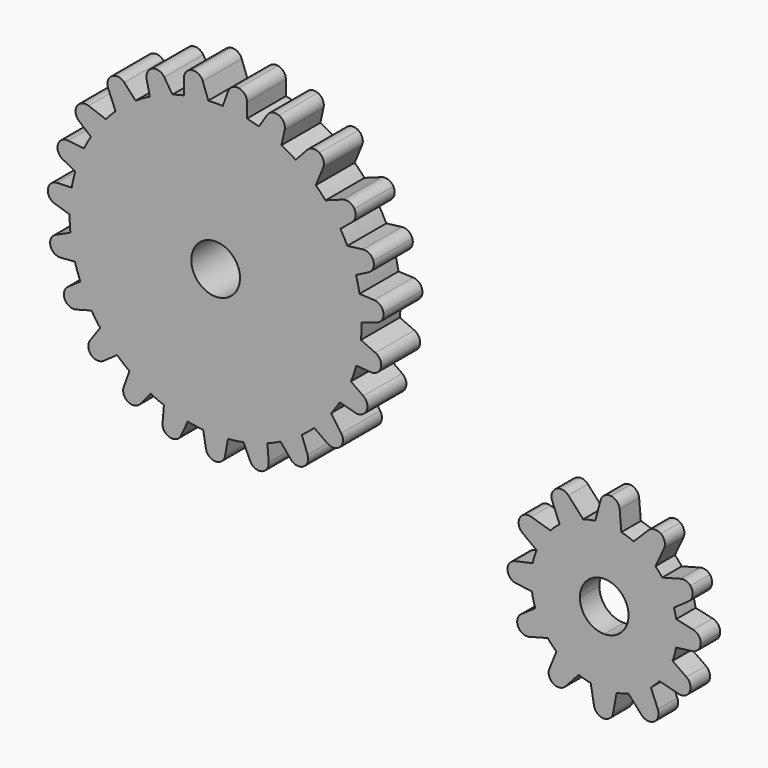
from build123d import *

# Parameters (mm, degrees)
F0_R     = 6.35
F1_DEPTH = 12.7
F3_DEPTH = 6.35


# Not quite as in the source:
# - ends of sketch curves that miss each other by under 0.0002 mm in the source are joined


with BuildPart() as f1:
    # F0 (on Front) → F1 (new body)
    with BuildSketch(Plane.XZ):
        with BuildLine():
            ThreePointArc((-34.9102419123, 17.5729671738), (-34.7547672057, 19.5550047024), (-34.7028952222, 21.5424539336))
            ThreePointArc((-34.7028952222, 21.5424539336), (-34.7029631236, 21.6143850332), (-34.7031668276, 21.6863158763))
            Line((-34.7031668276, 21.6863158763), (-37.8996429288, 20.6795870415))
            Line((-37.8996429288, 20.6795870415), (-38.8881478291, 28.2065023981))
            Line((-38.8881478291, 28.2065023981), (-35.2622454535, 28.047038082))
            ThreePointArc((-35.2622454535, 28.047038082), (-35.6708480799, 30.0759804631), (-36.1890238522, 32.0797412175))
            Line((-36.1890238522, 32.0797412175), (-39.5328523124, 30.3577733792))
            Line((-39.5328523124, 30.3577733792), (-41.7836899824, 37.6079683081))
            Line((-41.7836899824, 37.6079683081), (-38.4556661531, 38.0311729644))
            ThreePointArc((-38.4556661531, 38.0311729644), (-39.3128857232, 39.7091614987), (-40.2520180002, 41.3427163582))
            Line((-40.2520180002, 41.3427163582), (-42.874743432, 39.1419884157))
            Line((-42.874743432, 39.1419884157), (-46.67051729, 45.7164615917))
            Line((-46.67051729, 45.7164615917), (-44.1361986546, 46.6388781391))
            ThreePointArc((-44.1361986546, 46.6388781391), (-45.3794507172, 47.9917392071), (-46.6864795838, 49.2830890057))
            Line((-46.6864795838, 49.2830890057), (-47.6142884848, 47.0420555704))
            Line((-47.6142884848, 47.0420555704), (-54.0176456632, 51.1198752781))
            Line((-54.0176456632, 51.1198752781), (-51.920148722, 53.4096925747))
            ThreePointArc((-51.920148722, 53.4096925747), (-53.748897296, 54.5357132911), (-55.6381867093, 55.5569035347))
            Line((-55.6381867093, 55.5569035347), (-56.4261987077, 52.0361020119))
            Line((-56.4261987077, 52.0361020119), (-63.4339882382, 54.9554311505))
            Line((-63.4339882382, 54.9554311505), (-61.5269208328, 57.9356181485))
            ThreePointArc((-61.5269208328, 57.9356181485), (-63.0677548937, 58.3777229401), (-64.6258220077, 58.7546222881))
            Line((-64.6258220077, 58.7546222881), (-64.6258220077, 55.1074892599))
            Line((-64.6258220077, 55.1074892599), (-72.1020370557, 56.4257476864))
            Line((-72.1020370557, 56.4257476864), (-70.947701025, 59.5972598652))
            ThreePointArc((-70.947701025, 59.5972598652), (-72.8298646656, 59.6424443883), (-74.7119624515, 59.5945952966))
            Line((-74.7119624515, 59.5945952966), (-73.611945077, 56.5723223991))
            Line((-73.611945077, 56.5723223991), (-81.0892134905, 55.2538782358))
            Line((-81.0892134905, 55.2538782358), (-81.0892134905, 58.7304483613))
            ThreePointArc((-81.0892134905, 58.7304483613), (-82.5921118544, 58.3633887089), (-84.0788696115, 57.9356181485))
            Line((-84.0788696115, 57.9356181485), (-82.1718022061, 54.9554311505))
            Line((-82.1718022061, 54.9554311505), (-89.1795917366, 52.0361020119))
            Line((-89.1795917366, 52.0361020119), (-89.967603735, 55.5569035347))
            ThreePointArc((-89.967603735, 55.5569035347), (-91.8568931483, 54.5357132911), (-93.6856417223, 53.4096925747))
            Line((-93.6856417223, 53.4096925747), (-91.5881447811, 51.1198752781))
            Line((-91.5881447811, 51.1198752781), (-97.9915019595, 47.0420555704))
            Line((-97.9915019595, 47.0420555704), (-98.9193108605, 49.2830890057))
            ThreePointArc((-98.9193108605, 49.2830890057), (-100.2263397271, 47.9917392071), (-101.4695917897, 46.6388781391))
            Line((-101.4695917897, 46.6388781391), (-98.9352731543, 45.7164615917))
            Line((-98.9352731543, 45.7164615917), (-102.7310470123, 39.1419884157))
            Line((-102.7310470123, 39.1419884157), (-105.3537724441, 41.3427163582))
            ThreePointArc((-105.3537724441, 41.3427163582), (-106.2929047211, 39.7091614987), (-107.1501242912, 38.0311729644))
            Line((-107.1501242912, 38.0311729644), (-103.8221004619, 37.6079683081))
            Line((-103.8221004619, 37.6079683081), (-106.0729381319, 30.3577733792))
            Line((-106.0729381319, 30.3577733792), (-109.4167665921, 32.0797412175))
            ThreePointArc((-109.4167665921, 32.0797412175), (-109.9349423644, 30.0759804631), (-110.3435449908, 28.047038082))
            Line((-110.3435449908, 28.047038082), (-106.7176426152, 28.2065023981))
            Line((-106.7176426152, 28.2065023981), (-107.7061475155, 20.6795870415))
            Line((-107.7061475155, 20.6795870415), (-110.9026236167, 21.6863158763))
            ThreePointArc((-110.9026236167, 21.6863158763), (-110.854707645, 19.626841412), (-110.695548532, 17.5729671738))
            Line((-110.695548532, 17.5729671738), (-107.69785292, 18.9283214038))
            Line((-107.69785292, 18.9283214038), (-105.8189929076, 11.5729504562))
            Line((-105.8189929076, 11.5729504562), (-109.4987660128, 11.2943776791))
            ThreePointArc((-109.4987660128, 11.2943776791), (-108.8556105251, 9.221264085), (-108.0954397731, 7.1881410235))
            Line((-108.0954397731, 7.1881410235), (-105.2147046971, 9.2065173404))
            Line((-105.2147046971, 9.2065173404), (-102.0043529952, 2.3271831667))
            Line((-102.0043529952, 2.3271831667), (-105.1884891281, 1.4729918741))
            ThreePointArc((-105.1884891281, 1.4729918741), (-104.1087515023, -0.1728255389), (-102.9454542067, -1.760681861))
            Line((-102.9454542067, -1.760681861), (-101.2970690826, 0.5977276055))
            Line((-101.2970690826, 0.5977276055), (-95.9244653315, -4.7657344907))
            Line((-95.9244653315, -4.7657344907), (-98.5090591152, -6.5787682643))
            ThreePointArc((-98.5090591152, -6.5787682643), (-96.9341468953, -7.9413160541), (-95.2871392345, -9.2157770167))
            Line((-95.2871392345, -9.2157770167), (-94.2325988381, -6.3184510895))
            Line((-94.2325988381, -6.3184510895), (-87.658125662, -10.1142249475))
            Line((-87.658125662, -10.1142249475), (-89.734426864, -12.5886643643))
            ThreePointArc((-89.734426864, -12.5886643643), (-88.0370011642, -13.3793446476), (-86.3027767956, -14.0856697541))
            ThreePointArc((-86.3027767956, -14.0856697541), (-83.2302426255, -15.1028790043), (-80.0824621081, -15.8556463651))
            ThreePointArc((-80.0824621081, -15.8556463651), (-78.0770050025, -16.190737901), (-76.0565273803, -16.4183663655))
            ThreePointArc((-76.0565273803, -16.4183663655), (-72.8254583342, -16.5575393854), (-69.5942267157, -16.4221933902))
            ThreePointArc((-69.5942267157, -16.4221933902), (-67.551132252, -16.1938546525), (-65.5233283362, -15.8556463651))
            ThreePointArc((-65.5233283362, -15.8556463651), (-62.3755478188, -15.1028790043), (-59.3030136487, -14.0856697541))
            ThreePointArc((-59.3030136487, -14.0856697541), (-57.5687892801, -13.3793446476), (-55.8713635803, -12.5886643643))
            Line((-55.8713635803, -12.5886643643), (-57.9476647823, -10.1142249475))
            Line((-57.9476647823, -10.1142249475), (-51.3731916062, -6.3184510895))
            Line((-51.3731916062, -6.3184510895), (-50.3186512098, -9.2157770167))
            ThreePointArc((-50.3186512098, -9.2157770167), (-48.671643549, -7.9413160541), (-47.0967313291, -6.5787682643))
            Line((-47.0967313291, -6.5787682643), (-49.6813251128, -4.7657344907))
            Line((-49.6813251128, -4.7657344907), (-44.3087213617, 0.5977276055))
            Line((-44.3087213617, 0.5977276055), (-42.6603362376, -1.760681861))
            ThreePointArc((-42.6603362376, -1.760681861), (-41.497038942, -0.1728255389), (-40.4173013162, 1.4729918741))
            Line((-40.4173013162, 1.4729918741), (-43.6014374491, 2.3271831667))
            Line((-43.6014374491, 2.3271831667), (-40.3910857472, 9.2065173404))
            Line((-40.3910857472, 9.2065173404), (-37.5103506712, 7.1881410235))
            ThreePointArc((-37.5103506712, 7.1881410235), (-36.7501799192, 9.221264085), (-36.1070244315, 11.2943776791))
            Line((-36.1070244315, 11.2943776791), (-39.7867975367, 11.5729504562))
            Line((-39.7867975367, 11.5729504562), (-37.9079375243, 18.9283214038))
            Line((-37.9079375243, 18.9283214038), (-34.9102419123, 17.5729671738))
        make_face()
        with Locations((-72.8028952222, 21.5424539336)):
            Circle(F0_R, mode=Mode.SUBTRACT)
        with BuildLine():
            Line((-37.8996429288, 20.6795870415), (-34.7031668276, 21.6863158763))
            ThreePointArc((-34.7031668276, 21.6863158763), (-34.8492208425, 24.8784097313), (-35.2622454535, 28.047038082))
            Line((-35.2622454535, 28.047038082), (-38.8881478291, 28.2065023981))
            Line((-38.8881478291, 28.2065023981), (-37.8996429288, 20.6795870415))
        make_face()
        with BuildLine():
            ThreePointArc((-35.2622454535, 28.047038082), (-34.8492208425, 24.8784097313), (-34.7031668276, 21.6863158763))
            Line((-34.7031668276, 21.6863158763), (-30.7899816117, 22.9187719524))
            ThreePointArc((-30.7899816117, 22.9187719524), (-29.4112241553, 23.9760340856), (-29.0346296669, 25.6721920773))
            ThreePointArc((-29.0346296669, 25.6721920773), (-29.836410615, 27.2135926365), (-31.4414052089, 27.8790005528))
            Line((-31.4414052089, 27.8790005528), (-35.2622454535, 28.047038082))
        make_face()
        with BuildLine():
            Line((-31.1159582959, 15.857449985), (-34.9102419123, 17.5729671738))
            ThreePointArc((-34.9102419123, 17.5729671738), (-35.3767392162, 14.4085316873), (-36.1070244315, 11.2943776791))
            Line((-36.1070244315, 11.2943776791), (-32.3541248925, 11.0102689537))
            ThreePointArc((-32.3541248925, 11.0102689537), (-30.6812444479, 11.4795730766), (-29.7014065548, 12.9143877143))
            ThreePointArc((-29.7014065548, 12.9143877143), (-29.8730887811, 14.643345084), (-31.1159582959, 15.857449985))
        make_face()
        with BuildLine():
            ThreePointArc((-36.1070244315, 11.2943776791), (-35.3767392162, 14.4085316873), (-34.9102419123, 17.5729671738))
            Line((-34.9102419123, 17.5729671738), (-37.9079375243, 18.9283214038))
            Line((-37.9079375243, 18.9283214038), (-39.7867975367, 11.5729504562))
            Line((-39.7867975367, 11.5729504562), (-36.1070244315, 11.2943776791))
        make_face()
        with BuildLine():
            Line((-39.5328523124, 30.3577733792), (-36.1890238522, 32.0797412175))
            ThreePointArc((-36.1890238522, 32.0797412175), (-37.1977786118, 35.1028990281), (-38.4556661531, 38.0311729644))
            Line((-38.4556661531, 38.0311729644), (-41.7836899824, 37.6079683081))
            Line((-41.7836899824, 37.6079683081), (-39.5328523124, 30.3577733792))
        make_face()
        with BuildLine():
            ThreePointArc((-38.4556661531, 38.0311729644), (-37.1977786118, 35.1028990281), (-36.1890238522, 32.0797412175))
            Line((-36.1890238522, 32.0797412175), (-32.9059961539, 33.7703985511))
            ThreePointArc((-32.9059961539, 33.7703985511), (-31.7265399954, 35.0461957574), (-31.643090796, 36.7816529228))
            ThreePointArc((-31.643090796, 36.7816529228), (-32.6946947308, 38.1647283138), (-34.3892956008, 38.5482687065))
            Line((-34.3892956008, 38.5482687065), (-38.4556661531, 38.0311729644))
        make_face()
        with BuildLine():
            Line((-34.2864336087, 4.9293155241), (-37.5103506712, 7.1881410235))
            ThreePointArc((-37.5103506712, 7.1881410235), (-38.8433849386, 4.26930537), (-40.4173013162, 1.4729918741))
            Line((-40.4173013162, 1.4729918741), (-36.4020517039, 0.3958421817))
            ThreePointArc((-36.4020517039, 0.3958421817), (-34.6711564476, 0.5467625362), (-33.4422234889, 1.7749722596))
            ThreePointArc((-33.4422234889, 1.7749722596), (-33.2902851196, 3.5057764382), (-34.2864336087, 4.9293155241))
        make_face()
        with BuildLine():
            ThreePointArc((-40.4173013162, 1.4729918741), (-38.8433849386, 4.26930537), (-37.5103506712, 7.1881410235))
            Line((-37.5103506712, 7.1881410235), (-40.3910857472, 9.2065173404))
            Line((-40.3910857472, 9.2065173404), (-43.6014374491, 2.3271831667))
            Line((-43.6014374491, 2.3271831667), (-40.4173013162, 1.4729918741))
        make_face()
        with BuildLine():
            Line((-42.874743432, 39.1419884157), (-40.2520180002, 41.3427163582))
            ThreePointArc((-40.2520180002, 41.3427163582), (-42.0797741637, 44.0746493976), (-44.1361986546, 46.6388781391))
            Line((-44.1361986546, 46.6388781391), (-46.67051729, 45.7164615917))
            Line((-46.67051729, 45.7164615917), (-42.874743432, 39.1419884157))
        make_face()
        with BuildLine():
            ThreePointArc((-44.1361986546, 46.6388781391), (-42.0797741637, 44.0746493976), (-40.2520180002, 41.3427163582))
            Line((-40.2520180002, 41.3427163582), (-37.1646935203, 43.9332891906))
            ThreePointArc((-37.1646935203, 43.9332891906), (-36.2959623563, 45.4379757048), (-36.5976695233, 47.1490420761))
            ThreePointArc((-36.5976695233, 47.1490420761), (-37.9286418178, 48.2658594847), (-39.6661041459, 48.2658594847))
            Line((-39.6661041459, 48.2658594847), (-44.1361986546, 46.6388781391))
        make_face()
        with BuildLine():
            Line((-40.0385172453, -5.5118214706), (-42.6603362376, -1.760681861))
            ThreePointArc((-42.6603362376, -1.760681861), (-44.7748119678, -4.265229982), (-47.0967313291, -6.5787682643))
            Line((-47.0967313291, -6.5787682643), (-43.5790569647, -9.0463368499))
            ThreePointArc((-43.5790569647, -9.0463368499), (-41.9011807432, -9.4974540487), (-40.3258804416, -8.7645118264))
            ThreePointArc((-40.3258804416, -8.7645118264), (-39.5902580888, -7.1904635022), (-40.0385172453, -5.5118214706))
        make_face()
        with BuildLine():
            ThreePointArc((-47.0967313291, -6.5787682643), (-44.7748119678, -4.265229982), (-42.6603362376, -1.760681861))
            Line((-42.6603362376, -1.760681861), (-44.3087213617, 0.5977276055))
            Line((-44.3087213617, 0.5977276055), (-49.6813251128, -4.7657344907))
            Line((-49.6813251128, -4.7657344907), (-47.0967313291, -6.5787682643))
        make_face()
        with BuildLine():
            Line((-47.6142884848, 47.0420555704), (-46.6864795838, 49.2830890057))
            ThreePointArc((-46.6864795838, 49.2830890057), (-49.2129074162, 51.461051416), (-51.920148722, 53.4096925747))
            Line((-51.920148722, 53.4096925747), (-54.0176456632, 51.1198752781))
            Line((-54.0176456632, 51.1198752781), (-47.6142884848, 47.0420555704))
        make_face()
        with BuildLine():
            ThreePointArc((-51.920148722, 53.4096925747), (-49.2129074162, 51.461051416), (-46.6864795838, 49.2830890057))
            Line((-46.6864795838, 49.2830890057), (-44.7629890646, 53.9290959164))
            ThreePointArc((-44.7629890646, 53.9290959164), (-44.6875045379, 55.664917747), (-45.7454448011, 57.0431549331))
            ThreePointArc((-45.7454448011, 57.0431549331), (-47.4417860472, 57.4189138315), (-48.9827941123, 56.6163744339))
            Line((-48.9827941123, 56.6163744339), (-51.920148722, 53.4096925747))
        make_face()
        with BuildLine():
            Line((-48.8237937133, -13.3228642336), (-50.3186512098, -9.2157770167))
            ThreePointArc((-50.3186512098, -9.2157770167), (-53.0229828141, -11.0207932191), (-55.8713635803, -12.5886643643))
            Line((-55.8713635803, -12.5886643643), (-53.1563640074, -15.8242748592))
            ThreePointArc((-53.1563640074, -15.8242748592), (-51.6516774932, -16.6930060232), (-49.9406111219, -16.3912988562))
            ThreePointArc((-49.9406111219, -16.3912988562), (-48.8237937133, -15.0603265617), (-48.8237937133, -13.3228642336))
        make_face()
        with BuildLine():
            ThreePointArc((-55.8713635803, -12.5886643643), (-53.0229828141, -11.0207932191), (-50.3186512098, -9.2157770167))
            Line((-50.3186512098, -9.2157770167), (-51.3731916062, -6.3184510895))
            Line((-51.3731916062, -6.3184510895), (-57.9476647823, -10.1142249475))
            Line((-57.9476647823, -10.1142249475), (-55.8713635803, -12.5886643643))
        make_face()
        with BuildLine():
            Line((-56.4261987077, 52.0361020119), (-55.6381867093, 55.5569035347))
            ThreePointArc((-55.6381867093, 55.5569035347), (-58.5329028679, 56.8691763716), (-61.5269208328, 57.9356181485))
            Line((-61.5269208328, 57.9356181485), (-63.4339882382, 54.9554311505))
            Line((-63.4339882382, 54.9554311505), (-56.4261987077, 52.0361020119))
        make_face()
        with BuildLine():
            ThreePointArc((-61.5269208328, 57.9356181485), (-58.5329028679, 56.8691763716), (-55.6381867093, 55.5569035347))
            Line((-55.6381867093, 55.5569035347), (-54.7981656804, 59.3100790239))
            ThreePointArc((-54.7981656804, 59.3100790239), (-55.0214679679, 61.0331319627), (-56.3000845242, 62.2095311481))
            ThreePointArc((-56.3000845242, 62.2095311481), (-58.0357344825, 62.2888255062), (-59.4162909558, 61.2339135831))
            Line((-59.4162909558, 61.2339135831), (-61.5269208328, 57.9356181485))
        make_face()
        with BuildLine():
            Line((-58.9548245325, -18.3537802527), (-59.3030136487, -14.0856697541))
            ThreePointArc((-59.3030136487, -14.0856697541), (-62.3755478188, -15.1028790043), (-65.5233283362, -15.8556463651))
            Line((-65.5233283362, -15.8556463651), (-63.7946929451, -19.6202297071))
            ThreePointArc((-63.7946929451, -19.6202297071), (-62.5733513004, -20.8559885544), (-60.8434188448, -21.017571476))
            ThreePointArc((-60.8434188448, -21.017571476), (-59.4143522649, -20.0293725673), (-58.9548245325, -18.3537802527))
        make_face()
        with BuildLine():
            Line((-64.6258220077, 55.1074892599), (-64.6258220077, 58.7546222881))
            ThreePointArc((-64.6258220077, 58.7546222881), (-67.7690987546, 59.308455749), (-70.947701025, 59.5972598652))
            Line((-70.947701025, 59.5972598652), (-72.1020370557, 56.4257476864))
            Line((-72.1020370557, 56.4257476864), (-64.6258220077, 55.1074892599))
        make_face()
        with BuildLine():
            ThreePointArc((-70.947701025, 59.5972598652), (-67.7690987546, 59.308455749), (-64.6258220077, 58.7546222881))
            Line((-64.6258220077, 58.7546222881), (-64.6258220077, 62.561430037))
            ThreePointArc((-64.6258220077, 62.561430037), (-65.2200691221, 64.1941105656), (-66.7247556364, 65.0628417297))
            ThreePointArc((-66.7247556364, 65.0628417297), (-68.4358199059, 64.761134192), (-69.5526391627, 63.4301608305))
            Line((-69.5526391627, 63.4301608305), (-70.947701025, 59.5972598652))
        make_face()
        with BuildLine():
            Line((-70.3236177997, -20.5587757844), (-69.5942267157, -16.4221933902))
            ThreePointArc((-69.5942267157, -16.4221933902), (-72.8254583342, -16.5575393854), (-76.0565273803, -16.4183663655))
            Line((-76.0565273803, -16.4183663655), (-75.3264614886, -20.5587757844))
            ThreePointArc((-75.3264614886, -20.5587757844), (-74.4577303246, -22.0634622987), (-72.825049796, -22.6577094132))
            ThreePointArc((-72.825049796, -22.6577094132), (-71.1923489638, -22.0634622987), (-70.3236177997, -20.5587757844))
        make_face()
        with BuildLine():
            Line((-73.611945077, 56.5723223991), (-74.7119624515, 59.5945952966))
            ThreePointArc((-74.7119624515, 59.5945952966), (-77.9188661802, 59.297411769), (-81.0892134905, 58.7304483613))
            Line((-81.0892134905, 58.7304483613), (-81.0892134905, 55.2538782358))
            Line((-81.0892134905, 55.2538782358), (-73.611945077, 56.5723223991))
        make_face()
        with BuildLine():
            ThreePointArc((-81.0892134905, 58.7304483613), (-77.9188661802, 59.297411769), (-74.7119624515, 59.5945952966))
            Line((-74.7119624515, 59.5945952966), (-76.1623742386, 63.5795689305))
            ThreePointArc((-76.1623742386, 63.5795689305), (-77.2791934954, 64.9105422921), (-78.9902598666, 65.2122494591))
            ThreePointArc((-78.9902598666, 65.2122494591), (-80.494966376, 64.3435147694), (-81.0892134905, 62.7108342408))
            Line((-81.0892134905, 62.7108342408), (-81.0892134905, 58.7304483613))
        make_face()
        with BuildLine():
            Line((-81.8110974992, -19.6202297071), (-80.0824621081, -15.8556463651))
            ThreePointArc((-80.0824621081, -15.8556463651), (-83.2302426255, -15.1028790043), (-86.3027767956, -14.0856697541))
            Line((-86.3027767956, -14.0856697541), (-86.6509659118, -18.3537802527))
            ThreePointArc((-86.6509659118, -18.3537802527), (-86.1914381794, -20.0293725673), (-84.7623695349, -21.0175720162))
            ThreePointArc((-84.7623695349, -21.0175720162), (-83.0324391439, -20.8559885544), (-81.8110974992, -19.6202297071))
        make_face()
        with BuildLine():
            Line((-82.1718022061, 54.9554311505), (-84.0788696115, 57.9356181485))
            ThreePointArc((-84.0788696115, 57.9356181485), (-87.0728875764, 56.8691763716), (-89.967603735, 55.5569035347))
            Line((-89.967603735, 55.5569035347), (-89.1795917366, 52.0361020119))
            Line((-89.1795917366, 52.0361020119), (-82.1718022061, 54.9554311505))
        make_face()
        with BuildLine():
            ThreePointArc((-89.967603735, 55.5569035347), (-87.0728875764, 56.8691763716), (-84.0788696115, 57.9356181485))
            Line((-84.0788696115, 57.9356181485), (-86.1894994885, 61.2339135831))
            ThreePointArc((-86.1894994885, 61.2339135831), (-87.5700559618, 62.2888255062), (-89.3057078901, 62.2095303274))
            ThreePointArc((-89.3057078901, 62.2095303274), (-90.5843224764, 61.0331319627), (-90.8076247639, 59.3100790239))
            Line((-90.8076247639, 59.3100790239), (-89.967603735, 55.5569035347))
        make_face()
        with BuildLine():
            Line((-92.4494264369, -15.8242748592), (-89.734426864, -12.5886643643))
            ThreePointArc((-89.734426864, -12.5886643643), (-92.5828076302, -11.0207932191), (-95.2871392345, -9.2157770167))
            Line((-95.2871392345, -9.2157770167), (-96.781996731, -13.3228642336))
            ThreePointArc((-96.781996731, -13.3228642336), (-96.781996731, -15.0603265617), (-95.6651774742, -16.3912999233))
            ThreePointArc((-95.6651774742, -16.3912999233), (-93.9541129511, -16.6930060232), (-92.4494264369, -15.8242748592))
        make_face()
        with BuildLine():
            ThreePointArc((-95.2871392345, -9.2157770167), (-92.5828076302, -11.0207932191), (-89.734426864, -12.5886643643))
            Line((-89.734426864, -12.5886643643), (-87.658125662, -10.1142249475))
            Line((-87.658125662, -10.1142249475), (-94.2325988381, -6.3184510895))
            Line((-94.2325988381, -6.3184510895), (-95.2871392345, -9.2157770167))
        make_face()
        with BuildLine():
            Line((-91.5881447811, 51.1198752781), (-93.6856417223, 53.4096925747))
            ThreePointArc((-93.6856417223, 53.4096925747), (-96.3928830281, 51.461051416), (-98.9193108605, 49.2830890057))
            Line((-98.9193108605, 49.2830890057), (-97.9915019595, 47.0420555704))
            Line((-97.9915019595, 47.0420555704), (-91.5881447811, 51.1198752781))
        make_face()
        with BuildLine():
            ThreePointArc((-98.9193108605, 49.2830890057), (-96.3928830281, 51.461051416), (-93.6856417223, 53.4096925747))
            Line((-93.6856417223, 53.4096925747), (-96.622996332, 56.6163744339))
            ThreePointArc((-96.622996332, 56.6163744339), (-98.1640043971, 57.4189138315), (-99.8603474433, 57.0431537868))
            ThreePointArc((-99.8603474433, 57.0431537868), (-100.9182859064, 55.664917747), (-100.8428013797, 53.9290959164))
            Line((-100.8428013797, 53.9290959164), (-98.9193108605, 49.2830890057))
        make_face()
        with BuildLine():
            Line((-102.0267334796, -9.0463368499), (-98.5090591152, -6.5787682643))
            ThreePointArc((-98.5090591152, -6.5787682643), (-100.8309784765, -4.265229982), (-102.9454542067, -1.760681861))
            Line((-102.9454542067, -1.760681861), (-105.567273199, -5.5118214706))
            ThreePointArc((-105.567273199, -5.5118214706), (-106.0155323555, -7.1904635022), (-105.2799084923, -8.7645133341))
            ThreePointArc((-105.2799084923, -8.7645133341), (-103.7046097011, -9.4974540487), (-102.0267334796, -9.0463368499))
        make_face()
        with BuildLine():
            ThreePointArc((-102.9454542067, -1.760681861), (-100.8309784765, -4.265229982), (-98.5090591152, -6.5787682643))
            Line((-98.5090591152, -6.5787682643), (-95.9244653315, -4.7657344907))
            Line((-95.9244653315, -4.7657344907), (-101.2970690826, 0.5977276055))
            Line((-101.2970690826, 0.5977276055), (-102.9454542067, -1.760681861))
        make_face()
        with BuildLine():
            Line((-98.9352731543, 45.7164615917), (-101.4695917897, 46.6388781391))
            ThreePointArc((-101.4695917897, 46.6388781391), (-103.5260162806, 44.0746493976), (-105.3537724441, 41.3427163582))
            Line((-105.3537724441, 41.3427163582), (-102.7310470123, 39.1419884157))
            Line((-102.7310470123, 39.1419884157), (-98.9352731543, 45.7164615917))
        make_face()
        with BuildLine():
            ThreePointArc((-105.3537724441, 41.3427163582), (-103.5260162806, 44.0746493976), (-101.4695917897, 46.6388781391))
            Line((-101.4695917897, 46.6388781391), (-105.9396862984, 48.2658594847))
            ThreePointArc((-105.9396862984, 48.2658594847), (-107.6771486265, 48.2658594847), (-109.008121988, 47.1490402279))
            ThreePointArc((-109.008121988, 47.1490402279), (-109.309828088, 45.4379757048), (-108.441096924, 43.9332891906))
            Line((-108.441096924, 43.9332891906), (-105.3537724441, 41.3427163582))
        make_face()
        with BuildLine():
            Line((-109.2037387404, 0.3958421817), (-105.1884891281, 1.4729918741))
            ThreePointArc((-105.1884891281, 1.4729918741), (-106.7624055057, 4.26930537), (-108.0954397731, 7.1881410235))
            Line((-108.0954397731, 7.1881410235), (-111.3193568356, 4.9293155241))
            ThreePointArc((-111.3193568356, 4.9293155241), (-112.3155053247, 3.5057764382), (-112.1635660529, 1.7749703256))
            ThreePointArc((-112.1635660529, 1.7749703256), (-110.9346339967, 0.5467625362), (-109.2037387404, 0.3958421817))
        make_face()
        with BuildLine():
            ThreePointArc((-108.0954397731, 7.1881410235), (-106.7624055057, 4.26930537), (-105.1884891281, 1.4729918741))
            Line((-105.1884891281, 1.4729918741), (-102.0043529952, 2.3271831667))
            Line((-102.0043529952, 2.3271831667), (-105.2147046971, 9.2065173404))
            Line((-105.2147046971, 9.2065173404), (-108.0954397731, 7.1881410235))
        make_face()
        with BuildLine():
            Line((-103.8221004619, 37.6079683081), (-107.1501242912, 38.0311729644))
            ThreePointArc((-107.1501242912, 38.0311729644), (-108.4080118325, 35.1028990281), (-109.4167665921, 32.0797412175))
            Line((-109.4167665921, 32.0797412175), (-106.0729381319, 30.3577733792))
            Line((-106.0729381319, 30.3577733792), (-103.8221004619, 37.6079683081))
        make_face()
        with BuildLine():
            ThreePointArc((-109.4167665921, 32.0797412175), (-108.4080118325, 35.1028990281), (-107.1501242912, 38.0311729644))
            Line((-107.1501242912, 38.0311729644), (-111.2164948435, 38.5482687065))
            ThreePointArc((-111.2164948435, 38.5482687065), (-112.9110957135, 38.1647283138), (-113.962700281, 36.7816508846))
            ThreePointArc((-113.962700281, 36.7816508846), (-113.8792504489, 35.0461957574), (-112.6997942904, 33.7703985511))
            Line((-112.6997942904, 33.7703985511), (-109.4167665921, 32.0797412175))
        make_face()
        with BuildLine():
            Line((-113.2516655518, 11.0102689537), (-109.4987660128, 11.2943776791))
            ThreePointArc((-109.4987660128, 11.2943776791), (-110.2290512281, 14.4085316873), (-110.695548532, 17.5729671738))
            Line((-110.695548532, 17.5729671738), (-114.4898321484, 15.857449985))
            ThreePointArc((-114.4898321484, 15.857449985), (-115.7327016632, 14.643345084), (-115.9043833613, 12.9143856466))
            ThreePointArc((-115.9043833613, 12.9143856466), (-114.9245459964, 11.4795730766), (-113.2516655518, 11.0102689537))
        make_face()
        with BuildLine():
            ThreePointArc((-110.695548532, 17.5729671738), (-110.2290512281, 14.4085316873), (-109.4987660128, 11.2943776791))
            Line((-109.4987660128, 11.2943776791), (-105.8189929076, 11.5729504562))
            Line((-105.8189929076, 11.5729504562), (-107.69785292, 18.9283214038))
            Line((-107.69785292, 18.9283214038), (-110.695548532, 17.5729671738))
        make_face()
        with BuildLine():
            Line((-106.7176426152, 28.2065023981), (-110.3435449908, 28.047038082))
            ThreePointArc((-110.3435449908, 28.047038082), (-110.7565696018, 24.8784097313), (-110.9026236167, 21.6863158763))
            Line((-110.9026236167, 21.6863158763), (-107.7061475155, 20.6795870415))
            Line((-107.7061475155, 20.6795870415), (-106.7176426152, 28.2065023981))
        make_face()
        with BuildLine():
            ThreePointArc((-110.9026236167, 21.6863158763), (-110.7565696018, 24.8784097313), (-110.3435449908, 28.047038082))
            Line((-110.3435449908, 28.047038082), (-114.1643852354, 27.8790005528))
            ThreePointArc((-114.1643852354, 27.8790005528), (-115.7693798293, 27.2135926365), (-116.5711610553, 25.6721899613))
            ThreePointArc((-116.5711610553, 25.6721899613), (-116.194566289, 23.9760340856), (-114.8158088326, 22.9187719524))
            Line((-114.8158088326, 22.9187719524), (-110.9026236167, 21.6863158763))
        make_face()
    extrude(amount=F1_DEPTH)


with BuildPart() as f3:
    # F2 (on Front) → F3 (new body)
    with BuildSketch(Plane.XZ):
        with BuildLine():
            Line((39.2386662279, -27.221067247), (42.5388315106, -27.221067247))
            ThreePointArc((42.5388315106, -27.221067247), (42.4712083716, -25.6173625646), (42.2688190478, -24.0250434511))
            Line((42.2688190478, -24.0250434511), (39.4114386524, -23.3873699688))
            Line((39.4114386524, -23.3873699688), (39.2386662279, -27.221067247))
        make_face()
        with BuildLine():
            ThreePointArc((42.2688190478, -24.0250434511), (42.4712083716, -25.6173625646), (42.5388315106, -27.221067247))
            ThreePointArc((42.5388315106, -27.221067247), (42.4650633594, -28.8959179328), (42.2443302172, -30.5577974229))
            Line((42.2443302172, -30.5577974229), (46.4611879954, -30.0086556109))
            ThreePointArc((46.4611879954, -30.0086556109), (48.0034600385, -29.2085479391), (48.6706096692, -27.6042765431))
            ThreePointArc((48.6706096692, -27.6042765431), (48.1504700645, -25.9464999706), (46.6864204734, -25.0109070375))
            Line((46.6864204734, -25.0109070375), (42.2688190478, -24.0250434511))
        make_face()
        with BuildLine():
            ThreePointArc((42.2443302172, -30.5577974229), (42.4650633594, -28.8959179328), (42.5388315106, -27.221067247))
            Line((42.5388315106, -27.221067247), (39.2386662279, -27.221067247))
            Line((39.2386662279, -27.221067247), (39.0696588809, -30.9712201329))
            Line((39.0696588809, -30.9712201329), (42.2443302172, -30.5577974229))
        make_face()
        with BuildLine():
            Line((39.4114386524, -23.3873699688), (42.2688190478, -24.0250434511))
            ThreePointArc((42.2688190478, -24.0250434511), (42.0144891046, -22.7823162165), (41.6780192026, -21.5592697315))
            Line((41.6780192026, -21.5592697315), (39.3024932084, -23.217564621))
            Line((39.3024932084, -23.217564621), (36.1040258476, -16.3326969196))
            Line((36.1040258476, -16.3326969196), (38.6295404081, -15.6598634135))
            ThreePointArc((38.6295404081, -15.6598634135), (37.7754241148, -14.6196478126), (36.8499909676, -13.6423368953))
            Line((36.8499909676, -13.6423368953), (35.9346611892, -15.6009121348))
            Line((35.9346611892, -15.6009121348), (29.7197392831, -11.2412857258))
            Line((29.7197392831, -11.2412857258), (31.1736239134, -9.7898749262))
            ThreePointArc((31.1736239134, -9.7898749262), (29.590831745, -9.1747908128), (27.9595541548, -8.7030992419))
            Line((27.9595541548, -8.7030992419), (28.1592660179, -11.0084230784))
            Line((28.1592660179, -11.0084230784), (23.4888315106, -10.5958054377))
            Line((23.4888315106, -10.5958054377), (23.4888315106, -20.871067247))
            ThreePointArc((23.4888315106, -20.871067247), (27.9789595711, -22.7309391865), (29.8388315106, -27.221067247))
            Line((29.8388315106, -27.221067247), (39.2386662279, -27.221067247))
            Line((39.2386662279, -27.221067247), (39.4114386524, -23.3873699688))
        make_face()
        with BuildLine():
            ThreePointArc((41.3188553639, -33.9287307292), (41.8590768297, -32.2645369769), (42.2443302172, -30.5577974229))
            Line((42.2443302172, -30.5577974229), (39.0696588809, -30.9712201329))
            Line((39.0696588809, -30.9712201329), (39.2386662279, -27.221067247))
            Line((39.2386662279, -27.221067247), (29.8388315106, -27.221067247))
            ThreePointArc((29.8388315106, -27.221067247), (27.9789595711, -31.7111953075), (23.4888315106, -33.571067247))
            Line((23.4888315106, -33.571067247), (23.4888315106, -43.5467305829))
            Line((23.4888315106, -43.5467305829), (27.1324330255, -43.5498330739))
            Line((27.1324330255, -43.5498330739), (26.6984757495, -45.9987317413))
            ThreePointArc((26.6984757495, -45.9987317413), (28.2725179937, -45.6606671242), (29.8123945292, -45.1909044958))
            Line((29.8123945292, -45.1909044958), (28.2482940818, -43.4686322552))
            Line((28.2482940818, -43.4686322552), (34.6690657771, -39.4182881266))
            Line((34.6690657771, -39.4182881266), (35.6706278235, -41.8671021572))
            ThreePointArc((35.6706278235, -41.8671021572), (36.8326720529, -40.8168173029), (37.9045036776, -39.6746167801))
            Line((37.9045036776, -39.6746167801), (35.6145713384, -39.0631206306))
            Line((35.6145713384, -39.0631206306), (38.817038387, -32.1801124564))
            Line((38.817038387, -32.1801124564), (41.3188553639, -33.9287307292))
        make_face()
        with BuildLine():
            Line((39.3024932084, -23.217564621), (41.6780192026, -21.5592697315))
            ThreePointArc((41.6780192026, -21.5592697315), (40.4128159821, -18.475711359), (38.6295404081, -15.6598634135))
            Line((38.6295404081, -15.6598634135), (36.1040258476, -16.3326969196))
            Line((36.1040258476, -16.3326969196), (39.3024932084, -23.217564621))
        make_face()
        with BuildLine():
            ThreePointArc((38.6295404081, -15.6598634135), (40.4128159821, -18.475711359), (41.6780192026, -21.5592697315))
            Line((41.6780192026, -21.5592697315), (45.414522316, -18.9509109794))
            ThreePointArc((45.414522316, -18.9509109794), (46.5152556137, -17.179281474), (46.0014613402, -15.157821521))
            ThreePointArc((46.0014613402, -15.157821521), (44.7656661613, -14.3817317553), (43.306735988, -14.4137910486))
            Line((43.306735988, -14.4137910486), (38.6295404081, -15.6598634135))
        make_face()
        with BuildLine():
            Line((44.9265874631, -36.4503165729), (41.3188553639, -33.9287307292))
            ThreePointArc((41.3188553639, -33.9287307292), (39.8656452906, -36.9525866769), (37.9045036776, -39.6746167801))
            Line((37.9045036776, -39.6746167801), (42.8161653454, -40.9862110774))
            ThreePointArc((42.8161653454, -40.9862110774), (44.5468865364, -40.8333075107), (45.7744113691, -39.6036904457))
            ThreePointArc((45.7744113691, -39.6036904457), (45.9243664317, -37.8727133077), (44.9265874631, -36.4503165729))
        make_face()
        with BuildLine():
            ThreePointArc((37.9045036776, -39.6746167801), (39.8656452906, -36.9525866769), (41.3188553639, -33.9287307292))
            Line((41.3188553639, -33.9287307292), (38.817038387, -32.1801124564))
            Line((38.817038387, -32.1801124564), (35.6145713384, -39.0631206306))
            Line((35.6145713384, -39.0631206306), (37.9045036776, -39.6746167801))
        make_face()
        with BuildLine():
            ThreePointArc((17.1388315106, -27.221067247), (18.9987034501, -22.7309391865), (23.4888315106, -20.871067247))
            Line((23.4888315106, -20.871067247), (23.4888315106, -10.5958054377))
            Line((23.4888315106, -10.5958054377), (20.5971725602, -10.3403368102))
            Line((20.5971725602, -10.3403368102), (21.1413713275, -8.3162548785))
            ThreePointArc((21.1413713275, -8.3162548785), (19.5588049741, -8.5808582508), (18.0041193214, -8.9777004469))
            Line((18.0041193214, -8.9777004469), (19.1701500942, -10.2566665492))
            Line((19.1701500942, -10.2566665492), (12.7572274857, -14.3194267367))
            Line((12.7572274857, -14.3194267367), (11.8582732366, -12.1335686394))
            ThreePointArc((11.8582732366, -12.1335686394), (10.614507997, -13.1799029767), (9.4644620612, -14.3284506954))
            Line((9.4644620612, -14.3284506954), (11.5601212245, -14.9575260151))
            Line((11.5601212245, -14.9575260151), (8.1480631412, -21.7390786662))
            Line((8.1480631412, -21.7390786662), (5.8500100327, -20.0256189029))
            ThreePointArc((5.8500100327, -20.0256189029), (5.2671352493, -21.6647838346), (4.8362293039, -23.3502881368))
            Line((4.8362293039, -23.3502881368), (7.5154263103, -22.7523793363))
            Line((7.5154263103, -22.7523793363), (7.7168157233, -27.221067247))
            Line((7.7168157233, -27.221067247), (17.1388315106, -27.221067247))
        make_face()
        with BuildLine():
            Line((23.4888315106, -43.5467305829), (23.4888315106, -33.571067247))
            ThreePointArc((23.4888315106, -33.571067247), (18.9987034501, -31.7111953075), (17.1388315106, -27.221067247))
            Line((17.1388315106, -27.221067247), (7.7168157233, -27.221067247))
            Line((7.7168157233, -27.221067247), (7.8572060818, -30.3362295004))
            Line((7.8572060818, -30.3362295004), (4.6304188043, -29.9160199733))
            ThreePointArc((4.6304188043, -29.9160199733), (4.9769290868, -31.7168395558), (5.4949893261, -33.4759967782))
            Line((5.4949893261, -33.4759967782), (7.9777473395, -31.7406995645))
            Line((7.9777473395, -31.7406995645), (11.1802143881, -38.6237077387))
            Line((11.1802143881, -38.6237077387), (8.738077091, -39.2758482095))
            ThreePointArc((8.738077091, -39.2758482095), (9.8351581419, -40.5056336133), (11.0344231586, -41.6359974446))
            Line((11.0344231586, -41.6359974446), (12.0037950481, -39.2658881815))
            Line((12.0037950481, -39.2658881815), (18.4245667434, -43.3162323101))
            Line((18.4245667434, -43.3162323101), (16.8318087306, -45.0700601515))
            ThreePointArc((16.8318087306, -45.0700601515), (18.3781240614, -45.5727202888), (19.9616710875, -45.9416879458))
            Line((19.9616710875, -45.9416879458), (19.5408880616, -43.5433689477))
            Line((19.5408880616, -43.5433689477), (23.4888315106, -43.5467305829))
        make_face()
        with BuildLine():
            Line((35.9346611892, -15.6009121348), (36.8499909676, -13.6423368953))
            ThreePointArc((36.8499909676, -13.6423368953), (34.1866531686, -11.4584814257), (31.1736239134, -9.7898749262))
            Line((31.1736239134, -9.7898749262), (29.7197392831, -11.2412857258))
            Line((29.7197392831, -11.2412857258), (35.9346611892, -15.6009121348))
        make_face()
        with BuildLine():
            ThreePointArc((31.1736239134, -9.7898749262), (34.1866531686, -11.4584814257), (36.8499909676, -13.6423368953))
            Line((36.8499909676, -13.6423368953), (39.0905838365, -8.8480323525))
            ThreePointArc((39.0905838365, -8.8480323525), (39.2434874032, -7.1173111616), (38.2481321935, -5.6932172925))
            ThreePointArc((38.2481321935, -5.6932172925), (36.5702577192, -5.2421013192), (34.9949574176, -5.9750435416))
            Line((34.9949574176, -5.9750435416), (31.1736239134, -9.7898749262))
        make_face()
        with BuildLine():
            Line((37.4908283141, -46.317482956), (35.6706278235, -41.8671021572))
            ThreePointArc((35.6706278235, -41.8671021572), (32.8895759755, -43.7899689459), (29.8123945292, -45.1909044958))
            Line((29.8123945292, -45.1909044958), (33.2595471198, -48.9866550984))
            ThreePointArc((33.2595471198, -48.9866550984), (34.7971021868, -49.7957902894), (36.4950397773, -49.42730246))
            ThreePointArc((36.4950397773, -49.42730246), (37.5588742171, -48.0536122993), (37.4908283141, -46.317482956))
        make_face()
        with BuildLine():
            ThreePointArc((29.8123945292, -45.1909044958), (32.8895759755, -43.7899689459), (35.6706278235, -41.8671021572))
            Line((35.6706278235, -41.8671021572), (34.6690657771, -39.4182881266))
            Line((34.6690657771, -39.4182881266), (28.2482940818, -43.4686322552))
            Line((28.2482940818, -43.4686322552), (29.8123945292, -45.1909044958))
        make_face()
        with BuildLine():
            Line((20.5971725602, -10.3403368102), (23.4888315106, -10.5958054377))
            Line((23.4888315106, -10.5958054377), (23.4888315106, -8.171067247))
            ThreePointArc((23.4888315106, -8.171067247), (22.312858641, -8.2073988001), (21.1413713275, -8.3162548785))
            Line((21.1413713275, -8.3162548785), (20.5971725602, -10.3403368102))
        make_face()
        with BuildLine():
            Line((23.4888315106, -8.171067247), (23.4888315106, -10.5958054377))
            Line((23.4888315106, -10.5958054377), (28.1592660179, -11.0084230784))
            Line((28.1592660179, -11.0084230784), (27.9595541548, -8.7030992419))
            ThreePointArc((27.9595541548, -8.7030992419), (25.7399656139, -8.3045428504), (23.4888315106, -8.171067247))
        make_face()
        with BuildLine():
            Line((23.4888315106, -46.271067247), (23.4888315106, -43.5467305829))
            Line((23.4888315106, -43.5467305829), (19.5408880616, -43.5433689477))
            Line((19.5408880616, -43.5433689477), (19.9616710875, -45.9416879458))
            ThreePointArc((19.9616710875, -45.9416879458), (21.7175783261, -46.1885436779), (23.4888315106, -46.271067247))
        make_face()
        with BuildLine():
            Line((27.1324330255, -43.5498330739), (23.4888315106, -43.5467305829))
            Line((23.4888315106, -43.5467305829), (23.4888315106, -46.271067247))
            ThreePointArc((23.4888315106, -46.271067247), (25.0994201272, -46.2028612694), (26.6984757495, -45.9987317413))
            Line((26.6984757495, -45.9987317413), (27.1324330255, -43.5498330739))
        make_face()
        with BuildLine():
            Line((4.4388315106, -27.221067247), (7.7168157233, -27.221067247))
            Line((7.7168157233, -27.221067247), (7.5154263103, -22.7523793363))
            Line((7.5154263103, -22.7523793363), (4.8362293039, -23.3502881368))
            ThreePointArc((4.8362293039, -23.3502881368), (4.5384413822, -25.2755046082), (4.4388315106, -27.221067247))
        make_face()
        with BuildLine():
            Line((7.8572060818, -30.3362295004), (7.7168157233, -27.221067247))
            Line((7.7168157233, -27.221067247), (4.4388315106, -27.221067247))
            ThreePointArc((4.4388315106, -27.221067247), (4.4867886986, -28.5719443591), (4.6304188043, -29.9160199733))
            Line((4.6304188043, -29.9160199733), (7.8572060818, -30.3362295004))
        make_face()
        with BuildLine():
            ThreePointArc((21.1413713275, -8.3162548785), (22.312858641, -8.2073988001), (23.4888315106, -8.171067247))
            ThreePointArc((23.4888315106, -8.171067247), (25.7399656139, -8.3045428504), (27.9595541548, -8.7030992419))
            Line((27.9595541548, -8.7030992419), (27.5159353117, -3.5822963146))
            ThreePointArc((27.5159353117, -3.5822963146), (26.7829930894, -2.006996013), (25.2089432574, -1.2713721498))
            ThreePointArc((25.2089432574, -1.2713721498), (23.5303033517, -1.7196314941), (22.5325243831, -3.1420282289))
            Line((22.5325243831, -3.1420282289), (21.1413713275, -8.3162548785))
        make_face()
        with BuildLine():
            ThreePointArc((26.6984757495, -45.9987317413), (25.0994201272, -46.2028612694), (23.4888315106, -46.271067247))
            ThreePointArc((23.4888315106, -46.271067247), (21.7175783261, -46.1885436779), (19.9616710875, -45.9416879458))
            Line((19.9616710875, -45.9416879458), (20.829000294, -50.8851670916))
            ThreePointArc((20.829000294, -50.8851670916), (21.6964499177, -52.3905927762), (23.3286238591, -52.9862298862))
            ThreePointArc((23.3286238591, -52.9862298862), (24.9618076571, -52.3933731963), (25.8318197316, -50.8894269434))
            Line((25.8318197316, -50.8894269434), (26.6984757495, -45.9987317413))
        make_face()
        with BuildLine():
            ThreePointArc((4.6304188043, -29.9160199733), (4.4867886986, -28.5719443591), (4.4388315106, -27.221067247))
            ThreePointArc((4.4388315106, -27.221067247), (4.5384413822, -25.2755046082), (4.8362293039, -23.3502881368))
            Line((4.8362293039, -23.3502881368), (0.2404444893, -24.375916405))
            ThreePointArc((0.2404444893, -24.375916405), (-1.2236051018, -25.3115093381), (-1.7437446104, -26.9692880426))
            ThreePointArc((-1.7437446104, -26.9692880426), (-1.0765950758, -28.5735573066), (0.4656769673, -29.3736649783))
            Line((0.4656769673, -29.3736649783), (4.6304188043, -29.9160199733))
        make_face()
        with BuildLine():
            Line((19.1701500942, -10.2566665492), (18.0041193214, -8.9777004469))
            ThreePointArc((18.0041193214, -8.9777004469), (14.7869353512, -10.2746958587), (11.8582732366, -12.1335686394))
            Line((11.8582732366, -12.1335686394), (12.7572274857, -14.3194267367))
            Line((12.7572274857, -14.3194267367), (19.1701500942, -10.2566665492))
        make_face()
        with BuildLine():
            ThreePointArc((11.8582732366, -12.1335686394), (14.7869353512, -10.2746958587), (18.0041193214, -8.9777004469))
            Line((18.0041193214, -8.9777004469), (14.1482295374, -4.7483503791))
            ThreePointArc((14.1482295374, -4.7483503791), (12.6091117416, -3.9421917395), (10.9118903218, -4.3139642424))
            ThreePointArc((10.9118903218, -4.3139642424), (9.8507158457, -5.6897102597), (9.9221208823, -7.4257046901))
            Line((9.9221208823, -7.4257046901), (11.8582732366, -12.1335686394))
        make_face()
        with BuildLine():
            Line((13.4133137054, -48.8342551533), (16.8318087306, -45.0700601515))
            ThreePointArc((16.8318087306, -45.0700601515), (13.7800779013, -43.6113876634), (11.0344231586, -41.6359974446))
            Line((11.0344231586, -41.6359974446), (9.182032511, -46.1650830109))
            ThreePointArc((9.182032511, -46.1650830109), (9.1139866081, -47.9012123542), (10.1778228529, -49.2749036535))
            ThreePointArc((10.1778228529, -49.2749036535), (11.8757586383, -49.6433903444), (13.4133137054, -48.8342551533))
        make_face()
        with BuildLine():
            ThreePointArc((11.0344231586, -41.6359974446), (13.7800779013, -43.6113876634), (16.8318087306, -45.0700601515))
            Line((16.8318087306, -45.0700601515), (18.4245667434, -43.3162323101))
            Line((18.4245667434, -43.3162323101), (12.0037950481, -39.2658881815))
            Line((12.0037950481, -39.2658881815), (11.0344231586, -41.6359974446))
        make_face()
        with BuildLine():
            Line((2.1723525642, -17.2835072989), (5.8500100327, -20.0256189029))
            ThreePointArc((5.8500100327, -20.0256189029), (7.4030040118, -17.0157424761), (9.4644620612, -14.3284506954))
            Line((9.4644620612, -14.3284506954), (4.4208949337, -12.8144718679))
            ThreePointArc((4.4208949337, -12.8144718679), (2.6862984452, -12.9142233775), (1.4216394786, -14.1056145977))
            ThreePointArc((1.4216394786, -14.1056145977), (1.2186669786, -15.8311784294), (2.1723525642, -17.2835072989))
        make_face()
        with BuildLine():
            ThreePointArc((9.4644620612, -14.3284506954), (7.4030040118, -17.0157424761), (5.8500100327, -20.0256189029))
            Line((5.8500100327, -20.0256189029), (8.1480631412, -21.7390786662))
            Line((8.1480631412, -21.7390786662), (11.5601212245, -14.9575260151))
            Line((11.5601212245, -14.9575260151), (9.4644620612, -14.3284506954))
        make_face()
        with BuildLine():
            Line((7.9777473395, -31.7406995645), (5.4949893261, -33.4759967782))
            ThreePointArc((5.4949893261, -33.4759967782), (6.8616934271, -36.5184205883), (8.738077091, -39.2758482095))
            Line((8.738077091, -39.2758482095), (11.1802143881, -38.6237077387))
            Line((11.1802143881, -38.6237077387), (7.9777473395, -31.7406995645))
        make_face()
        with BuildLine():
            ThreePointArc((8.738077091, -39.2758482095), (6.8616934271, -36.5184205883), (5.4949893261, -33.4759967782))
            Line((5.4949893261, -33.4759967782), (1.8681982634, -36.010903681))
            ThreePointArc((1.8681982634, -36.010903681), (0.8704192948, -37.4333004159), (1.0203752576, -39.1642794887))
            ThreePointArc((1.0203752576, -39.1642794887), (2.2478991901, -40.3938946188), (3.9786203811, -40.5467981855))
            Line((3.9786203811, -40.5467981855), (8.738077091, -39.2758482095))
        make_face()
    extrude(amount=F3_DEPTH)


solid = Compound([f1.part, f3.part])
